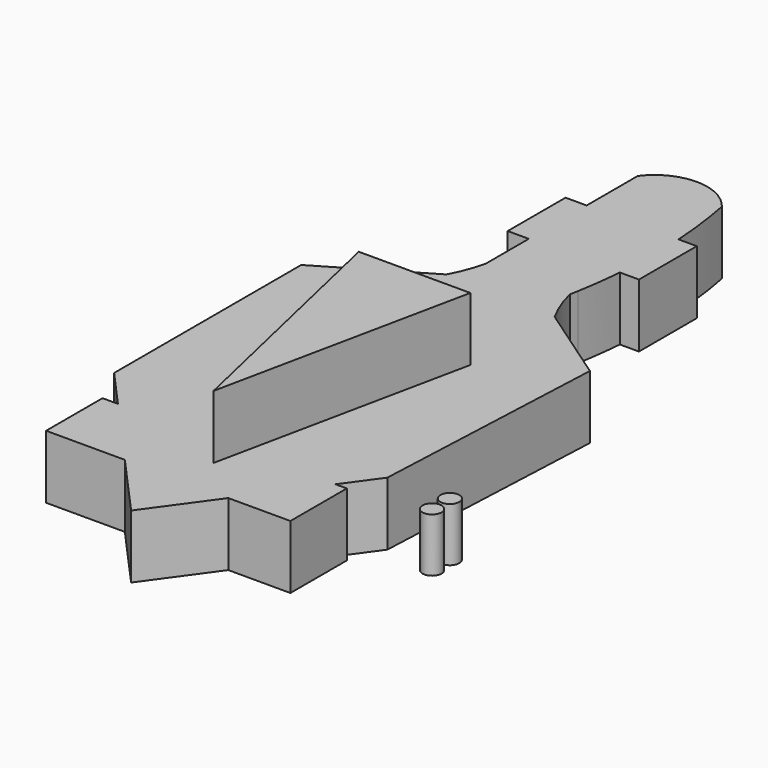
from build123d import *

# Parameters (mm, degrees)
F0_DEPTH  = 25.4
F15_DEPTH = 25.4
F6_DEPTH  = 25.4
F7_W      = 52.5711476803
F7_H      = 28.9547294378
F8_DEPTH  = 25.4
F9_R      = 3.7869940918
F10_DEPTH = 21.59
F18_R     = 3.8055561705
F11_DEPTH = 21.59
F19_W     = 97.8483408689
F19_H     = 28.2483398914
F12_DEPTH = 25.4


# Not quite as in the source:
# - the program builds the solid bodies; features that only make, move or delete a surface that nothing else refers to are left out


with BuildPart() as f0:
    # F13 (on Top) → F0 (new body)
    with BuildSketch(Plane.XY):
        with BuildLine():
            ThreePointArc((16.2997245058, 3.3815672953), (19.3231299232, 39.8030258746), (15.6745165586, 76.1671736836))
            ThreePointArc((15.6745165586, 76.1671736836), (-1.1504060771, 84.3494571695), (-17.8354382515, 75.8855640888))
            Line((-17.8354382515, 75.8855640888), (-17.8354382515, 0))
            ThreePointArc((-17.8354382515, 0), (-29.0742141651, -22.5080976821), (-49.6557429433, -36.9761735201))
            ThreePointArc((-49.6557429433, -36.9761735201), (-53.2002321262, -80.6407257915), (-49.6557429433, -124.3052780628))
            ThreePointArc((-49.6557429433, -124.3052780628), (-28.552755811, -158.7517318324), (0, -187.3285472393))
            ThreePointArc((0, -187.3285472393), (23.5369802762, -157.5088719546), (41.433095932, -123.9987015724))
            ThreePointArc((41.433095932, -123.9987015724), (43.4568628888, -79.9188986421), (41.433095932, -35.8390957117))
            ThreePointArc((41.433095932, -35.8390957117), (25.0609068527, -20.4299941844), (15.6745165586, 0))
            ThreePointArc((15.6745165586, 0), (15.9943820769, 1.6894410822), (16.2997245058, 3.3815672953))
        make_face()
    extrude(amount=F0_DEPTH)

    # F14 (on face) → F15 (join)
    with BuildSketch(Plane.XY.offset(25.4)):
        Polygon((21.2603222236, -56.7732304335), (-23.4202891588, -56.7732304335), (0, -158.7517318324), align=None)
    extrude(amount=F15_DEPTH)

    # F5 (on Top) → F6 (join)
    with BuildSketch(Plane.XY):
        Polygon((0, 0), (-62.3636394739, -36.9194597006), (-62.3636394739, -130.5717527866), (0, -200.0146508217), (48.659875989, -132.5382590294), (52.991092205, -36.5707874298), align=None)
    extrude(amount=F6_DEPTH)

    # F7 (on Top) → F8 (join)
    with BuildSketch(Plane.XY):
        with Locations((0, 35.8452573419)):
            Rectangle(F7_W, F7_H)
    extrude(amount=F8_DEPTH)

    # F19 (on Top) → F12 (join)
    with BuildSketch(Plane.XY):
        with Locations((-5.5963620543, -160.3068858385)):
            Rectangle(F19_W, F19_H)
    extrude(amount=F12_DEPTH)


with BuildPart() as f10:
    # F9 (on Top) → F10 (new body)
    with BuildSketch(Plane.XY):
        with Locations((68.1670159101, -125.6581246853)):
            Circle(F9_R)
    extrude(amount=F10_DEPTH)


with BuildPart() as f11:
    # F18 (on Top) → F11 (new body)
    with BuildSketch(Plane.XY):
        with Locations((68.230509758, -134.652659297)):
            Circle(F18_R)
    extrude(amount=F11_DEPTH)


solid = Compound([f0.part, f10.part, f11.part])
